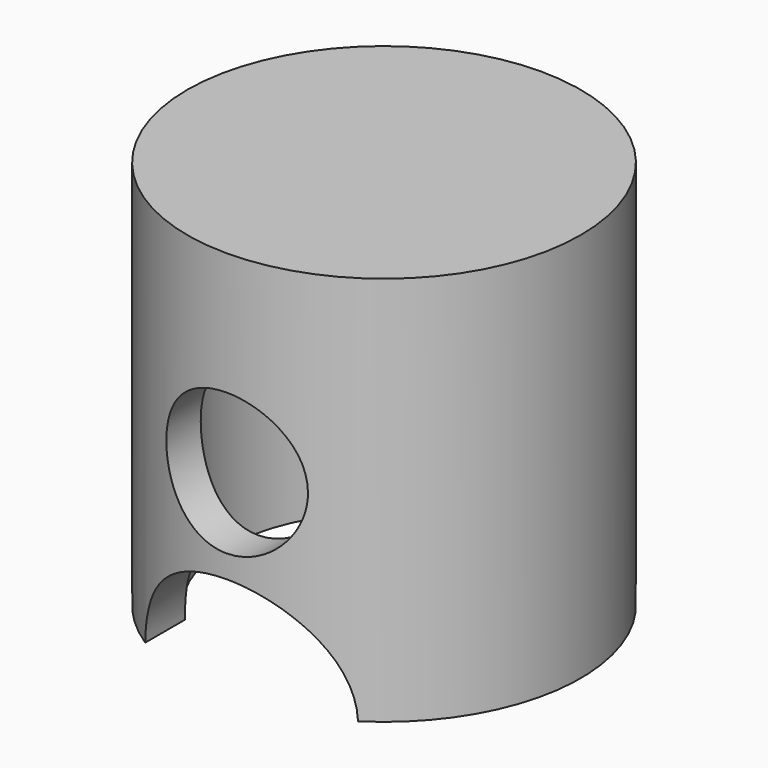
from build123d import *

# Parameters (mm, degrees)
F3_R          = 3.599766951
F4_DEPTH      = 10.001
F4_DEPTH_BACK = 10.001
F6_DEPTH      = 10.0010001
F6_DEPTH_BACK = 10.0010001


with BuildPart() as f2:
    # F0 (on Right) → F2 (revolve)
    with BuildSketch(Plane.YZ):
        Polygon((0, 18), (0, 20), (-10, 20), (-10, 0.1677852448), (-8, 0.1677852448), (-8, 18), align=None)
    revolve(axis=Axis((0, 0, 9.9367983639), (0, 0, -1)))

    # F3 (on Front) → F4 (cut, two sides)
    with BuildSketch(Plane.XZ) as f4_sk:
        with Locations((0, 10.1677852448)):
            Circle(F3_R)
    extrude(amount=-F4_DEPTH, mode=Mode.SUBTRACT)
    extrude(f4_sk.sketch, amount=F4_DEPTH_BACK, mode=Mode.SUBTRACT)

    # F5 (on Front) → F6 (cut, two sides)
    with BuildSketch(Plane.XZ) as f6_sk:
        with BuildLine():
            Line((-5.4118316221, 0), (5.4118316221, 0))
            ThreePointArc((5.4118316221, 0), (0, 5.4118316221), (-5.4118316221, 0))
        make_face()
    extrude(amount=-F6_DEPTH, mode=Mode.SUBTRACT)
    extrude(f6_sk.sketch, amount=F6_DEPTH_BACK, mode=Mode.SUBTRACT)


solid = f2.part
